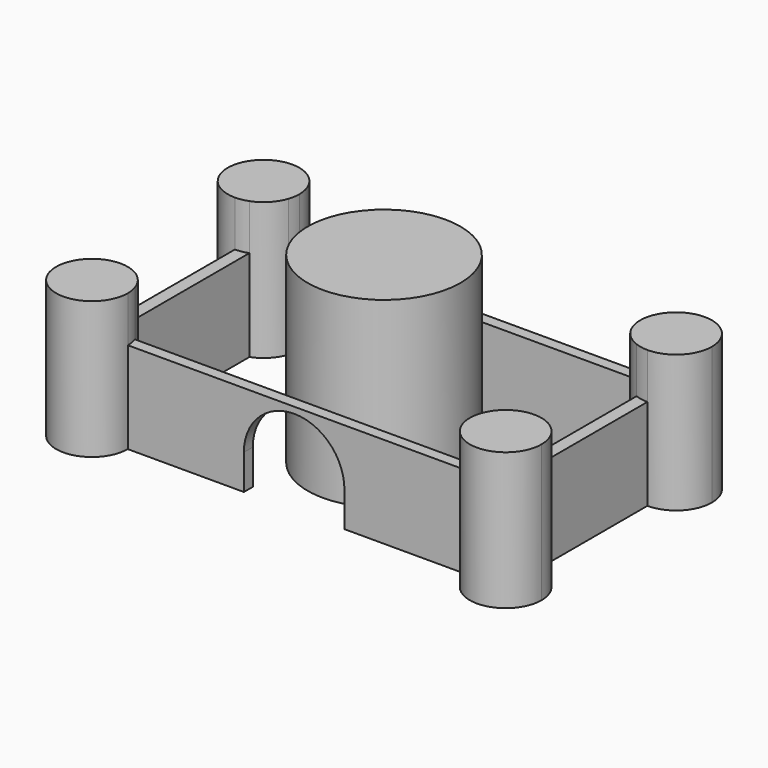
from build123d import *

# Parameters (mm, degrees)
F1_DEPTH = 25.4
F2_DEPTH = 38.1
F0_R     = 21.2222684157
F3_DEPTH = 50.8
F5_DEPTH = 25.4


# Not quite as in the source:
# - a feature of the source that left no trace in its solid (it failed there, or was rolled back) is left out


with BuildPart() as f1:
    # F0 (on Top) → F1 (new body)
    with BuildSketch(Plane.XY):
        with BuildLine():
            Line((57.2681427002, -19.2034440821), (57.2681427002, 19.7960699943))
            ThreePointArc((57.2681427002, 19.7960699943), (55.4813658991, 19.9619755545), (53.7534877658, 20.4462617803))
            Line((53.7534877658, 20.4462617803), (53.7534877658, -19.7758921918))
            ThreePointArc((53.7534877658, -19.7758921918), (55.4849853919, -19.3310808749), (57.2681427002, -19.2034440821))
        make_face()
    extrude(amount=F1_DEPTH)


with BuildPart() as f1b:
    # F0 (on Top) → F1, piece 2 (new body)
    with BuildSketch(Plane.XY):
        with BuildLine():
            ThreePointArc((-47.3303807535, -29.7702029347), (-47.330380765, -29.7706825659), (-47.3303807997, -29.771162197))
            Line((-47.3303807997, -29.771162197), (47.1581171171, -29.771162197))
            ThreePointArc((47.1581171171, -29.771162197), (47.1828392876, -28.209007874), (47.4519053251, -26.6700014472))
            Line((47.4519053251, -26.6700014472), (-47.8259358741, -26.6700014472))
            ThreePointArc((-47.8259358741, -26.6700014472), (-47.4550509459, -28.2004239582), (-47.3303807535, -29.7702029347))
        make_face()
    extrude(amount=F1_DEPTH)

    # F4 (on face) → F5 (cut)
    with BuildSketch(Plane.XZ.offset(29.771162197)):
        with BuildLine():
            Line((-15.0923253968, 0), (0, 0))
            Line((0, 0), (12.8181409091, 0))
            Line((12.8181409091, 0), (12.8181409091, 9.716976434))
            ThreePointArc((12.8181409091, 9.716976434), (-1.1370922439, 23.6722095869), (-15.0923253968, 9.716976434))
            Line((-15.0923253968, 9.716976434), (-15.0923253968, 0))
        make_face()
    extrude(amount=-F5_DEPTH, mode=Mode.SUBTRACT)


with BuildPart() as f1c:
    # F0 (on Top) → F1, piece 3 (new body)
    with BuildSketch(Plane.XY):
        with BuildLine():
            ThreePointArc((-53.7534877658, 20.4676737388), (-55.4817610377, 19.9876793123), (-57.2681427002, 19.8259273179))
            Line((-57.2681427002, 19.8259273179), (-57.2681427002, -19.8249708633))
            ThreePointArc((-57.2681427002, -19.8249708633), (-55.4816289767, -19.9881117126), (-53.7534877658, -20.469541018))
            Line((-53.7534877658, -20.469541018), (-53.7534877658, 20.4676737388))
        make_face()
    extrude(amount=F1_DEPTH)


with BuildPart() as f1d:
    # F0 (on Top) → F1, piece 4 (new body)
    with BuildSketch(Plane.XY):
        with BuildLine():
            ThreePointArc((47.8313635292, 26.6700014472), (47.4652042143, 28.2012835622), (47.345293281, 29.771162197))
            Line((47.345293281, 29.771162197), (-47.3229078211, 29.771162197))
            ThreePointArc((-47.3229078211, 29.771162197), (-47.4476577038, 28.2008847583), (-47.8187777055, 26.6700014472))
            Line((-47.8187777055, 26.6700014472), (47.8313635292, 26.6700014472))
        make_face()
    extrude(amount=F1_DEPTH)


with BuildPart() as f2:
    # F0 (on Top) → F2 (new body)
    with BuildSketch(Plane.XY):
        with BuildLine():
            ThreePointArc((67.2357181452, 29.7412797809), (57.305424491, 39.6865034364), (47.345293281, 29.771162197))
            ThreePointArc((47.345293281, 29.771162197), (47.4652042143, 28.2012835622), (47.8313635292, 26.6700014472))
            ThreePointArc((47.8313635292, 26.6700014472), (50.0857288168, 22.8856827883), (53.7534877658, 20.4462617803))
            ThreePointArc((53.7534877658, 20.4462617803), (55.4813658991, 19.9619755545), (57.2681427002, 19.7960699943))
            ThreePointArc((57.2681427002, 19.7960699943), (64.314923266, 22.7010426053), (67.2357181452, 29.7412797809))
        make_face()
    extrude(amount=F2_DEPTH)


with BuildPart() as f2b:
    # F0 (on Top) → F2, piece 2 (new body)
    with BuildSketch(Plane.XY):
        with BuildLine():
            ThreePointArc((67.0289794348, -29.1469693184), (64.1809827389, -22.1801259176), (57.2681427002, -19.2034440821))
            ThreePointArc((57.2681427002, -19.2034440821), (55.4849853919, -19.3310808749), (53.7534877658, -19.7758921918))
            ThreePointArc((53.7534877658, -19.7758921918), (49.7430246375, -22.4371609842), (47.4519053251, -26.6700014472))
            ThreePointArc((47.4519053251, -26.6700014472), (47.1828392876, -28.209007874), (47.1581171171, -29.771162197))
            ThreePointArc((47.1581171171, -29.771162197), (57.3959949366, -39.0873011287), (67.0289794348, -29.1469693184))
        make_face()
    extrude(amount=F2_DEPTH)


with BuildPart() as f2c:
    # F0 (on Top) → F2, piece 3 (new body)
    with BuildSketch(Plane.XY):
        with BuildLine():
            ThreePointArc((-53.7534877658, -20.469541018), (-55.4816289767, -19.9881117126), (-57.2681427002, -19.8249708633))
            ThreePointArc((-57.2681427002, -19.8249708633), (-64.3109392552, -36.7995640952), (-47.3303807997, -29.771162197))
            ThreePointArc((-47.3303807997, -29.771162197), (-47.330380765, -29.7706825659), (-47.3303807535, -29.7702029347))
            ThreePointArc((-47.3303807535, -29.7702029347), (-47.4550509459, -28.2004239582), (-47.8259358741, -26.6700014472))
            ThreePointArc((-47.8259358741, -26.6700014472), (-50.0868483078, -22.8978437219), (-53.7534877658, -20.469541018))
        make_face()
    extrude(amount=F2_DEPTH)


with BuildPart() as f2d:
    # F0 (on Top) → F2, piece 4 (new body)
    with BuildSketch(Plane.XY):
        with BuildLine():
            ThreePointArc((-47.8187777055, 26.6700014472), (-47.4476577038, 28.2008847583), (-47.3229078211, 29.771162197))
            ThreePointArc((-47.3229078211, 29.771162197), (-64.3004857237, 36.8035052205), (-57.2681427002, 19.8259273179))
            ThreePointArc((-57.2681427002, 19.8259273179), (-55.4817610377, 19.9876793123), (-53.7534877658, 20.4676737388))
            ThreePointArc((-53.7534877658, 20.4676737388), (-50.0824854281, 22.8955512155), (-47.8187777055, 26.6700014472))
        make_face()
    extrude(amount=F2_DEPTH)


with BuildPart() as f3:
    # F0 (on Top) → F3 (new body)
    with BuildSketch(Plane.XY):
        Circle(F0_R)
    extrude(amount=F3_DEPTH)


solid = Compound([f1.part, f1b.part, f1c.part, f1d.part, f2.part, f2b.part, f2c.part, f2d.part, f3.part])
